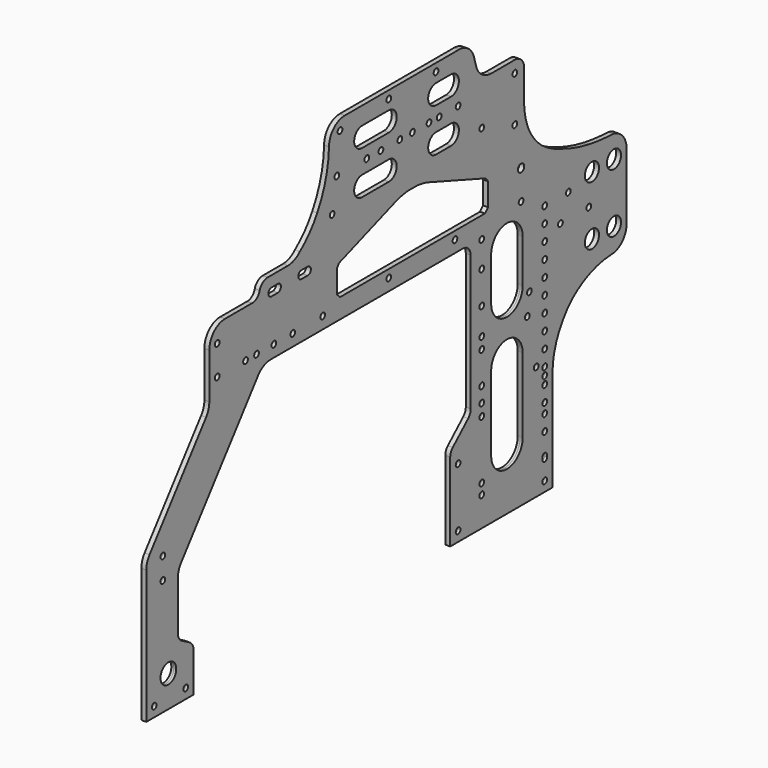
from build123d import *

# Parameters (mm, degrees)
F0_R     = 1.5
F0_R_2   = 5
F0_R_3   = 4.5
F0_R_4   = 2
F1_DEPTH = 1.25


# Not quite as in the source:
# - ends of sketch curves that miss each other by under 0.0002 mm in the source are joined


with BuildPart() as f1:
    # F0 (on Right) → F1 (new body, symmetric)
    with BuildSketch(Plane.YZ):
        with BuildLine():
            Line((105.495477, -110), (105.495477, -58))
            ThreePointArc((105.495477, -58), (105.8241359148, -54.1028914723), (106.4954774522, -50.2500000996))
            ThreePointArc((106.4954774522, -50.2500000996), (110.8327711884, -39.6668658213), (117.9954770131, -30.7500000141))
            ThreePointArc((117.9954770131, -30.7500000141), (129.4294199149, -23.8243949833), (142.4954769758, -20.999999486))
            ThreePointArc((142.4954769758, -20.999999486), (149.7106529517, -18.0361473468), (152.4954764033, -10.7500000256))
            Line((152.4954764033, -10.7500000256), (152.495477, 23))
            ThreePointArc((152.495477, 23), (149.9000389985, 29.2303976573), (143.9954771405, 32.5000008159))
            ThreePointArc((143.9954771405, 32.5000008159), (136.4707242857, 33.0024728567), (128.9954770501, 34.0000002997))
            ThreePointArc((128.9954770501, 34.0000002997), (119.4621390383, 36.2102114949), (110.245476888, 39.4999997355))
            ThreePointArc((110.245476888, 39.4999997355), (104.3929795082, 42.0734421956), (98.995477348, 45.5000004661))
            ThreePointArc((98.995477348, 45.5000004661), (94.1691726191, 50.2834678821), (90.495476792, 55.9999998965))
            ThreePointArc((90.495476792, 55.9999998965), (88.4052185086, 61.8524353772), (87.4954766996, 67.9999999853))
            Line((87.4954766996, 67.9999999853), (87.495477, 85))
            ThreePointArc((87.495477, 85), (85.7381176871, 89.2426406871), (81.495477, 91))
            Line((81.495477, 91), (72.495477, 91))
            Line((72.495477, 91), (66.511288, 91))
            ThreePointArc((66.511288, 91), (60.5032021513, 93.0060707763), (56.905645391, 98.2194191132))
            Line((56.905645391, 98.2194191132), (55.585309, 102.780581))
            ThreePointArc((55.585309, 102.780581), (51.9877518487, 107.9939292237), (45.979666, 110))
            Line((45.979666, 110), (-2.004523, 110))
            Line((-2.004523, 110), (-26.504523, 110))
            ThreePointArc((-26.504523, 110), (-33.5755908119, 107.0710678119), (-36.504523, 100))
            ThreePointArc((-36.504523, 100), (-38.5885297772, 86.2784924794), (-44.0045227356, 73.4999998465))
            ThreePointArc((-44.0045227356, 73.4999998465), (-48.8666319251, 66.5746626172), (-55.0045232099, 60.7500002708))
            ThreePointArc((-55.0045232099, 60.7500002708), (-58.4479074584, 58.4174256151), (-62.5045229891, 57.4999996968))
            Line((-62.5045229891, 57.4999996968), (-75.504523, 57.5))
            ThreePointArc((-75.504523, 57.5), (-78.6053948, 56.4261624), (-80.5045227218, 53.7499999118))
            ThreePointArc((-80.5045227218, 53.7499999118), (-82.3141729218, 50.9545333087), (-85.5045229812, 50.0000003033))
            Line((-85.5045229812, 50.0000003033), (-102.504523, 50))
            ThreePointArc((-102.504523, 50), (-109.5755908119, 47.0710678119), (-112.504523, 40))
            Line((-112.504523, 40), (-112.504523, 16.892597))
            ThreePointArc((-112.504523, 16.892597), (-113.0346610986, 13.6798543137), (-114.5688661137, 10.8077510872))
            Line((-114.5688661137, 10.8077510872), (-150.44018, -35.974451))
            ThreePointArc((-150.44018, -35.974451), (-151.9743849014, -38.8465543137), (-152.504523, -42.059297))
            Line((-152.504523, -42.059297), (-152.504523, -110))
            Line((-152.504523, -110), (-122.504523, -110))
            Line((-122.504523, -110), (-122.504523, -89.956356))
            ThreePointArc((-122.504523, -89.956356), (-123.2005730203, -87.4115545201), (-125.0949288289, -85.5752766889))
            Line((-125.0949288289, -85.5752766889), (-129.914117, -82.924723))
            ThreePointArc((-129.914117, -82.924723), (-131.8084729797, -81.0884454799), (-132.504523, -78.543644))
            Line((-132.504523, -78.543644), (-132.504523, -53.889733))
            ThreePointArc((-132.504523, -53.889733), (-131.9752097928, -50.6794227856), (-130.4433046654, -47.8089644903))
            Line((-130.4433046654, -47.8089644903), (-81.506483, 16.080775))
            ThreePointArc((-81.506483, 16.080775), (-77.9944610281, 18.9668223611), (-73.567713, 20.000006))
            Line((-73.567713, 20.000006), (48.495477, 20))
            ThreePointArc((48.495477, 20), (52.0310109059, 18.5355339059), (53.495477, 15))
            Line((53.495477, 15), (53.495477, -53.702577))
            ThreePointArc((53.495477, -53.702577), (53.0729214073, -55.7142933563), (51.8766759207, -57.3859849137))
            Line((51.8766759207, -57.3859849137), (42.114278, -66.347415))
            ThreePointArc((42.114278, -66.347415), (40.9180325927, -68.0191066437), (40.495477, -70.030823))
            Line((40.495477, -70.030823), (40.495477, -110))
            Line((40.495477, -110), (105.495477, -110))
        make_face()
        with Locations((-147.504523, -105)):
            Circle(F0_R, mode=Mode.SUBTRACT)
        with Locations((-127.504523, -105)):
            Circle(F0_R, mode=Mode.SUBTRACT)
        with Locations((-138.504523, -94)):
            Circle(F0_R_2, mode=Mode.SUBTRACT)
        with Locations((-142.004523, -51)):
            Circle(F0_R, mode=Mode.SUBTRACT)
        with Locations((-142.004523, -40)):
            Circle(F0_R, mode=Mode.SUBTRACT)
        with Locations((45.495477, -105)):
            Circle(F0_R, mode=Mode.SUBTRACT)
        with Locations((60.495477, -95)):
            Circle(F0_R, mode=Mode.SUBTRACT)
        with Locations((60.495477, -89.75)):
            Circle(F0_R, mode=Mode.SUBTRACT)
        with Locations((45.495477, -75)):
            Circle(F0_R, mode=Mode.SUBTRACT)
        with Locations((60.495477, -60)):
            Circle(F0_R, mode=Mode.SUBTRACT)
        with Locations((100.495477, -105)):
            Circle(F0_R, mode=Mode.SUBTRACT)
        with BuildLine():
            Line((98.995477, -95), (98.995477, -94))
            ThreePointArc((98.995477, -94), (99.4348168282, -92.9393398282), (100.495477, -92.5))
            ThreePointArc((100.495477, -92.5), (101.5561371718, -92.9393398282), (101.995477, -94))
            Line((101.995477, -94), (101.995477, -95))
            ThreePointArc((101.995477, -95), (101.5561371718, -96.0606601718), (100.495477, -96.5))
            ThreePointArc((100.495477, -96.5), (99.4348168282, -96.0606601718), (98.995477, -95))
        make_face(mode=Mode.SUBTRACT)
        with Locations((100.495477, -83)):
            Circle(F0_R, mode=Mode.SUBTRACT)
        with Locations((100.495477, -75)):
            Circle(F0_R, mode=Mode.SUBTRACT)
        with Locations((100.495477, -70)):
            Circle(F0_R, mode=Mode.SUBTRACT)
        with BuildLine():
            Line((66.495477, -80), (66.495477, -42))
            ThreePointArc((66.495477, -42), (69.4244091881, -34.9289321881), (76.495477, -32))
            ThreePointArc((76.495477, -32), (83.5665448119, -34.9289321881), (86.495477, -42))
            Line((86.495477, -42), (86.495477, -80))
            ThreePointArc((86.495477, -80), (83.5665448119, -87.0710678119), (76.495477, -90))
            ThreePointArc((76.495477, -90), (69.4244091881, -87.0710678119), (66.495477, -80))
        make_face(mode=Mode.SUBTRACT)
        with Locations((100.495477, -62)):
            Circle(F0_R, mode=Mode.SUBTRACT)
        with Locations((100.495477, -58)):
            Circle(F0_R, mode=Mode.SUBTRACT)
        with Locations((60.495477, -54)):
            Circle(F0_R, mode=Mode.SUBTRACT)
        with Locations((60.495477, -46.25)):
            Circle(F0_R, mode=Mode.SUBTRACT)
        with Locations((60.495477, -30)):
            Circle(F0_R, mode=Mode.SUBTRACT)
        with Locations((60.495477, -24.25)):
            Circle(F0_R, mode=Mode.SUBTRACT)
        with Locations((60.495477, -10.5)):
            Circle(F0_R, mode=Mode.SUBTRACT)
        with Locations((95.115862, -51.870676)):
            Circle(F0_R, mode=Mode.SUBTRACT)
        with Locations((100.495477, -54)):
            Circle(F0_R, mode=Mode.SUBTRACT)
        with Locations((100.495477, -46)):
            Circle(F0_R, mode=Mode.SUBTRACT)
        with Locations((100.495477, -38)):
            Circle(F0_R, mode=Mode.SUBTRACT)
        with Locations((100.495477, -30)):
            Circle(F0_R, mode=Mode.SUBTRACT)
        with Locations((89.495477, -27)):
            Circle(F0_R, mode=Mode.SUBTRACT)
        with Locations((90.745477, -16.5)):
            Circle(F0_R, mode=Mode.SUBTRACT)
        with Locations((100.495477, -22)):
            Circle(F0_R, mode=Mode.SUBTRACT)
        with Locations((100.495477, -14)):
            Circle(F0_R, mode=Mode.SUBTRACT)
        with BuildLine():
            Line((66.495477, -12), (66.495477, 10))
            ThreePointArc((66.495477, 10), (69.4244091881, 17.0710678119), (76.495477, 20))
            ThreePointArc((76.495477, 20), (83.5665448119, 17.0710678119), (86.495477, 10))
            Line((86.495477, 10), (86.495477, -12))
            ThreePointArc((86.495477, -12), (83.5665448119, -19.0710678119), (76.495477, -22))
            ThreePointArc((76.495477, -22), (69.4244091881, -19.0710678119), (66.495477, -12))
        make_face(mode=Mode.SUBTRACT)
        with Locations((100.495477, -6)):
            Circle(F0_R, mode=Mode.SUBTRACT)
        with Locations((130.495477, -9)):
            Circle(F0_R_3, mode=Mode.SUBTRACT)
        with Locations((144.495477, -9)):
            Circle(F0_R_3, mode=Mode.SUBTRACT)
        with Locations((-107.504523, 26)):
            Circle(F0_R, mode=Mode.SUBTRACT)
        with Locations((-89.504523, 26)):
            Circle(F0_R, mode=Mode.SUBTRACT)
        with Locations((-82.504523, 26)):
            Circle(F0_R, mode=Mode.SUBTRACT)
        with Locations((-107.504523, 41)):
            Circle(F0_R, mode=Mode.SUBTRACT)
        with Locations((-71.504523, 26)):
            Circle(F0_R, mode=Mode.SUBTRACT)
        with Locations((-59.504523, 26)):
            Circle(F0_R, mode=Mode.SUBTRACT)
        with Locations((-40.504523, 26)):
            Circle(F0_R, mode=Mode.SUBTRACT)
        with BuildLine():
            ThreePointArc((-73.004523, 48), (-74.4187365624, 48.5857864376), (-75.004523, 50))
            ThreePointArc((-75.004523, 50), (-74.4187365624, 51.4142135624), (-73.004523, 52))
            Line((-73.004523, 52), (-69.004523, 52))
            ThreePointArc((-69.004523, 52), (-67.5903094376, 51.4142135624), (-67.004523, 50))
            ThreePointArc((-67.004523, 50), (-67.5903094376, 48.5857864376), (-69.004523, 48))
            Line((-69.004523, 48), (-73.004523, 48))
        make_face(mode=Mode.SUBTRACT)
        with BuildLine():
            ThreePointArc((-54.004523, 48), (-55.4187365624, 48.5857864376), (-56.004523, 50))
            ThreePointArc((-56.004523, 50), (-55.4187365624, 51.4142135624), (-54.004523, 52))
            Line((-54.004523, 52), (-50.004523, 52))
            ThreePointArc((-50.004523, 52), (-48.5903094376, 51.4142135624), (-48.004523, 50))
            ThreePointArc((-48.004523, 50), (-48.5903094376, 48.5857864376), (-50.004523, 48))
            Line((-50.004523, 48), (-54.004523, 48))
        make_face(mode=Mode.SUBTRACT)
        with Locations((-34.504523, 69)):
            Circle(F0_R, mode=Mode.SUBTRACT)
        with BuildLine():
            ThreePointArc((-15.504523, 69), (-19.0400569059, 70.4644660941), (-20.504523, 74))
            ThreePointArc((-20.504523, 74), (-19.0400569059, 77.5355339059), (-15.504523, 79))
            Line((-15.504523, 79), (1.495477, 79))
            ThreePointArc((1.495477, 79), (5.0310109059, 77.5355339059), (6.495477, 74))
            ThreePointArc((6.495477, 74), (5.0310109059, 70.4644660941), (1.495477, 69))
            Line((1.495477, 69), (-15.504523, 69))
        make_face(mode=Mode.SUBTRACT)
        with Locations((-31.504523, 85)):
            Circle(F0_R, mode=Mode.SUBTRACT)
        with Locations((-12.504523, 85)):
            Circle(F0_R, mode=Mode.SUBTRACT)
        with Locations((-3.504523, 85)):
            Circle(F0_R, mode=Mode.SUBTRACT)
        with BuildLine():
            ThreePointArc((-15.504523, 91), (-19.0400569059, 92.4644660941), (-20.504523, 96))
            ThreePointArc((-20.504523, 96), (-19.0400569059, 99.5355339059), (-15.504523, 101))
            Line((-15.504523, 101), (1.495477, 101))
            ThreePointArc((1.495477, 101), (5.0310109059, 99.5355339059), (6.495477, 96))
            ThreePointArc((6.495477, 96), (5.0310109059, 92.4644660941), (1.495477, 91))
            Line((1.495477, 91), (-15.504523, 91))
        make_face(mode=Mode.SUBTRACT)
        with Locations((-29.504523, 104.5)):
            Circle(F0_R, mode=Mode.SUBTRACT)
        with Locations((1.495477, 26)):
            Circle(F0_R, mode=Mode.SUBTRACT)
        with Locations((60.495477, 6)):
            Circle(F0_R, mode=Mode.SUBTRACT)
        with Locations((43.495477, 26)):
            Circle(F0_R, mode=Mode.SUBTRACT)
        with Locations((60.495477, 19.25)):
            Circle(F0_R, mode=Mode.SUBTRACT)
        Polygon((7.885515, 59.067871), (13.266897, 60), (19.724057, 60), (25.105439, 59.067871), (63.16815, 45.474045), (64.495477, 43.590562), (64.495477, 32), (62.495477, 30), (-29.504523, 30), (-31.504523, 32), (-31.504523, 43.590562), (-30.177196, 45.474045), align=None, mode=Mode.SUBTRACT)
        with Locations((100.495477, 2)):
            Circle(F0_R, mode=Mode.SUBTRACT)
        with Locations((110.495477, 6)):
            Circle(F0_R, mode=Mode.SUBTRACT)
        with Locations((100.495477, 10)):
            Circle(F0_R, mode=Mode.SUBTRACT)
        with Locations((85.495477, 26)):
            Circle(F0_R, mode=Mode.SUBTRACT)
        with Locations((100.495477, 18)):
            Circle(F0_R, mode=Mode.SUBTRACT)
        with Locations((128.495477, 6)):
            Circle(F0_R, mode=Mode.SUBTRACT)
        with Locations((115.495477, 18)):
            Circle(F0_R, mode=Mode.SUBTRACT)
        with Locations((130.495477, 21)):
            Circle(F0_R_3, mode=Mode.SUBTRACT)
        with Locations((144.495477, 21)):
            Circle(F0_R_3, mode=Mode.SUBTRACT)
        with Locations((85.495477, 41)):
            Circle(F0_R_4, mode=Mode.SUBTRACT)
        with BuildLine():
            ThreePointArc((31.495477, 69), (27.9599430941, 70.4644660941), (26.495477, 74))
            ThreePointArc((26.495477, 74), (27.9599430941, 77.5355339059), (31.495477, 79))
            Line((31.495477, 79), (40.995477, 79))
            ThreePointArc((40.995477, 79), (44.5310109059, 77.5355339059), (45.995477, 74))
            ThreePointArc((45.995477, 74), (44.5310109059, 70.4644660941), (40.995477, 69))
            Line((40.995477, 69), (31.495477, 69))
        make_face(mode=Mode.SUBTRACT)
        with Locations((60.495477, 69)):
            Circle(F0_R, mode=Mode.SUBTRACT)
        with Locations((8.495477, 85)):
            Circle(F0_R, mode=Mode.SUBTRACT)
        with Locations((16.495477, 85)):
            Circle(F0_R, mode=Mode.SUBTRACT)
        with Locations((26.995477, 85)):
            Circle(F0_R, mode=Mode.SUBTRACT)
        with Locations((33.495477, 85)):
            Circle(F0_R, mode=Mode.SUBTRACT)
        with BuildLine():
            ThreePointArc((31.495477, 91), (27.9599430941, 92.4644660941), (26.495477, 96))
            ThreePointArc((26.495477, 96), (27.9599430941, 99.5355339059), (31.495477, 101))
            Line((31.495477, 101), (40.995477, 101))
            ThreePointArc((40.995477, 101), (44.5310109059, 99.5355339059), (45.995477, 96))
            ThreePointArc((45.995477, 96), (44.5310109059, 92.4644660941), (40.995477, 91))
            Line((40.995477, 91), (31.495477, 91))
        make_face(mode=Mode.SUBTRACT)
        with Locations((1.495477, 106)):
            Circle(F0_R, mode=Mode.SUBTRACT)
        with Locations((31.495477, 106)):
            Circle(F0_R, mode=Mode.SUBTRACT)
        with Locations((45.495477, 85)):
            Circle(F0_R, mode=Mode.SUBTRACT)
        with Locations((81.495477, 62)):
            Circle(F0_R, mode=Mode.SUBTRACT)
        with Locations((81.495477, 85)):
            Circle(F0_R, mode=Mode.SUBTRACT)
    extrude(amount=F1_DEPTH, both=True)


solid = f1.part
